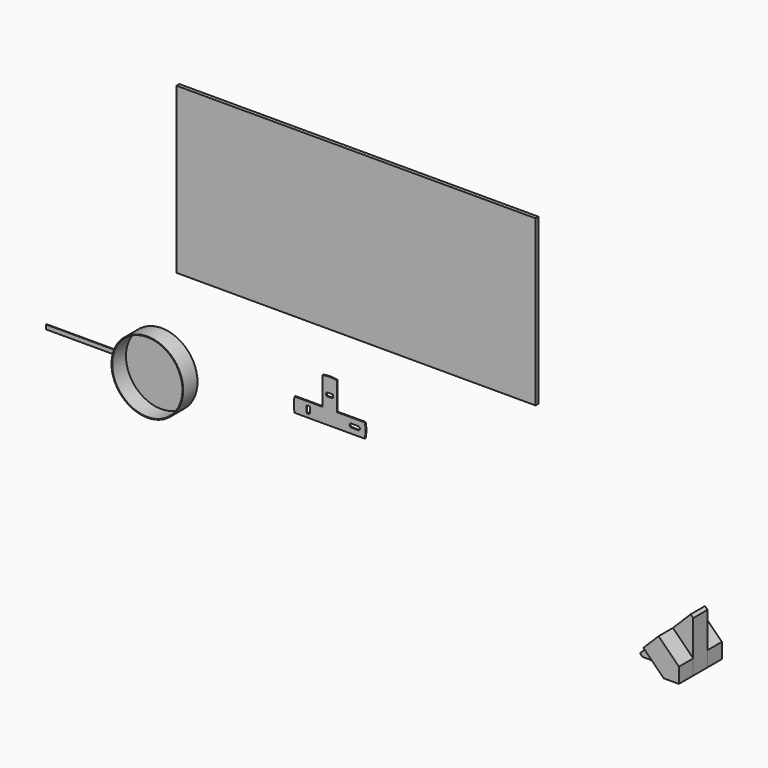
from build123d import *

# Parameters (mm, degrees)
F0_R      = 50
F1_DEPTH  = 25
F2_T      = -1
F3_DEPTH  = 1
F5_DEPTH  = 1.5
F4_W      = 500.6877612323
F4_H      = 229.7869026661
F7_DEPTH  = 5
F8_DEPTH  = 25
F9_W      = 25
F9_H      = 100
F11_DEPTH = 5
F13_DEPTH = 25
F15_DEPTH = 25


# Not quite as in the source:
# - the program builds the solid bodies; features that only make, move or delete a surface that nothing else refers to are left out


with BuildPart() as f1:
    # F0 (on Front) → F1 (new body)
    with BuildSketch(Plane.XZ):
        with Locations((-2.272e-07, 0.3450742583)):
            Circle(F0_R)
    extrude(amount=F1_DEPTH)

    # F2
    f2_openings = [f1.faces().sort_by_distance(p)[0] for p in [
        (0, -25, 0.345074),
    ]]
    offset(amount=F2_T, openings=f2_openings)


with BuildPart() as f3:
    # F0 (on Front) → F3 (new body)
    with BuildSketch(Plane.XZ):
        Polygon((-60.5894945183, -3.1098189969), (-60.5480098743, 2.8901810031), (-160.4069377537, 2.8901810031), (-160.3654531097, -3.1098189969), align=None)
    extrude(amount=F3_DEPTH)


with BuildPart() as f5:
    # F4 (on Front) → F5 (new body)
    with BuildSketch(Plane.XZ):
        with BuildLine():
            Line((225.5204433411, 27.5586571583), (186.5306484854, 27.5586571583))
            ThreePointArc((186.5306484854, 27.5586571583), (185.5204433411, 17.5586571583), (186.5306484854, 7.5586571583))
            Line((186.5306484854, 7.5586571583), (284.5102381967, 7.5586571583))
            ThreePointArc((284.5102381967, 7.5586571583), (285.2672509913, 12.533209058), (285.5204433411, 17.5586571583))
            ThreePointArc((285.5204433411, 17.5586571583), (285.2672509913, 22.5841052585), (284.5102381967, 27.5586571583))
            Line((284.5102381967, 27.5586571583), (245.5204433411, 27.5586571583))
            Line((245.5204433411, 27.5586571583), (245.5204433411, 66.5484520139))
            ThreePointArc((245.5204433411, 66.5484520139), (235.5204433411, 67.5586571583), (225.5204433411, 66.5484520139))
            Line((225.5204433411, 66.5484520139), (225.5204433411, 27.5586571583))
        make_face()
        with BuildLine():
            ThreePointArc((203.0204433411, 20.5586571583), (203.6062297787, 21.9728707206), (205.0204433411, 22.5586571583))
            Line((205.0204433411, 22.5586571583), (205.5204433411, 22.5586571583))
            Line((205.5204433411, 22.5586571583), (206.0204433411, 22.5586571583))
            ThreePointArc((206.0204433411, 22.5586571583), (207.4346569034, 21.9728707206), (208.0204433411, 20.5586571583))
            Line((208.0204433411, 20.5586571583), (208.0204433411, 14.5586571583))
            ThreePointArc((208.0204433411, 14.5586571583), (207.4346569034, 13.1444435959), (206.0204433411, 12.5586571583))
            Line((206.0204433411, 12.5586571583), (205.5204433411, 12.5586571583))
            Line((205.5204433411, 12.5586571583), (205.0204433411, 12.5586571583))
            ThreePointArc((205.0204433411, 12.5586571583), (203.6062297787, 13.1444435959), (203.0204433411, 14.5586571583))
            Line((203.0204433411, 14.5586571583), (203.0204433411, 20.5586571583))
        make_face(mode=Mode.SUBTRACT)
        with BuildLine():
            ThreePointArc((275.5204433411, 20.0586571583), (276.9346569034, 19.4728707206), (277.5204433411, 18.0586571583))
            Line((277.5204433411, 18.0586571583), (277.5204433411, 17.5586571583))
            Line((277.5204433411, 17.5586571583), (277.5204433411, 17.0586571583))
            ThreePointArc((277.5204433411, 17.0586571583), (276.9346569034, 15.6444435959), (275.5204433411, 15.0586571583))
            Line((275.5204433411, 15.0586571583), (265.5204433411, 15.0586571583))
            ThreePointArc((265.5204433411, 15.0586571583), (264.1062297787, 15.6444435959), (263.5204433411, 17.0586571583))
            Line((263.5204433411, 17.0586571583), (263.5204433411, 17.5586571583))
            Line((263.5204433411, 17.5586571583), (263.5204433411, 18.0586571583))
            ThreePointArc((263.5204433411, 18.0586571583), (264.1062297787, 19.4728707206), (265.5204433411, 20.0586571583))
            Line((265.5204433411, 20.0586571583), (275.5204433411, 20.0586571583))
        make_face(mode=Mode.SUBTRACT)
        with BuildLine():
            Line((232.5204433411, 47.5586571583), (238.5204433411, 47.5586571583))
            ThreePointArc((238.5204433411, 47.5586571583), (239.9346569034, 46.9728707206), (240.5204433411, 45.5586571583))
            Line((240.5204433411, 45.5586571583), (240.5204433411, 45.0586571583))
            Line((240.5204433411, 45.0586571583), (240.5204433411, 44.5586571583))
            ThreePointArc((240.5204433411, 44.5586571583), (239.9346569034, 43.1444435959), (238.5204433411, 42.5586571583))
            Line((238.5204433411, 42.5586571583), (232.5204433411, 42.5586571583))
            ThreePointArc((232.5204433411, 42.5586571583), (231.1062297787, 43.1444435959), (230.5204433411, 44.5586571583))
            Line((230.5204433411, 44.5586571583), (230.5204433411, 45.0586571583))
            Line((230.5204433411, 45.0586571583), (230.5204433411, 45.5586571583))
            ThreePointArc((230.5204433411, 45.5586571583), (231.1062297787, 46.9728707206), (232.5204433411, 47.5586571583))
        make_face(mode=Mode.SUBTRACT)
    extrude(amount=F5_DEPTH)


with BuildPart() as f7:
    # F4 (on Front) → F7 (new body)
    with BuildSketch(Plane.XZ):
        with Locations((275.1347804442, 243.0963665247)):
            Rectangle(F4_W, F4_H)
    extrude(amount=F7_DEPTH)


with BuildPart() as f8:
    # F4 (on Front) → F8 (new body)
    with BuildSketch(Plane.XZ):
        Polygon((761.4211719814, -118.7199804553), (761.4211719814, -48.0093023367), (690.7104938628, -118.7199804553), align=None)
    extrude(amount=F8_DEPTH)

    # F9 (on face) → F11 (join)
    with BuildSketch(Plane(origin=(404.7152371591, 0, -404.7152371591), x_dir=(0, -1, 0), z_dir=(-0.7071067812, 0, 0.7071067812))):
        with Locations((12.5, 454.4583708048)):
            Rectangle(F9_W, F9_H)
    extrude(amount=F11_DEPTH)


with BuildPart() as f13:
    # F12 (on Front) → F13 (new body)
    with BuildSketch(Plane.XZ):
        Polygon((761.4211719814, -118.7199804553), (761.4211719814, -97.5067770197), (733.136900734, -69.2225057723), (711.9236972984, -90.4357092079), (740.2079685458, -118.7199804553), align=None)
    extrude(amount=-F13_DEPTH)


with BuildPart() as f15:
    # F14 (on face) → F15 (new body)
    with BuildSketch(Plane.XZ.offset(25)):
        Polygon((761.4211719814, -118.7199804553), (761.4211719814, -97.5067770197), (733.136900734, -69.2225057723), (711.9236972984, -90.4357092079), (740.2079685458, -118.7199804553), align=None)
    extrude(amount=F15_DEPTH)


solid = Compound([f1.part, f3.part, f5.part, f7.part, f8.part, f13.part, f15.part])
